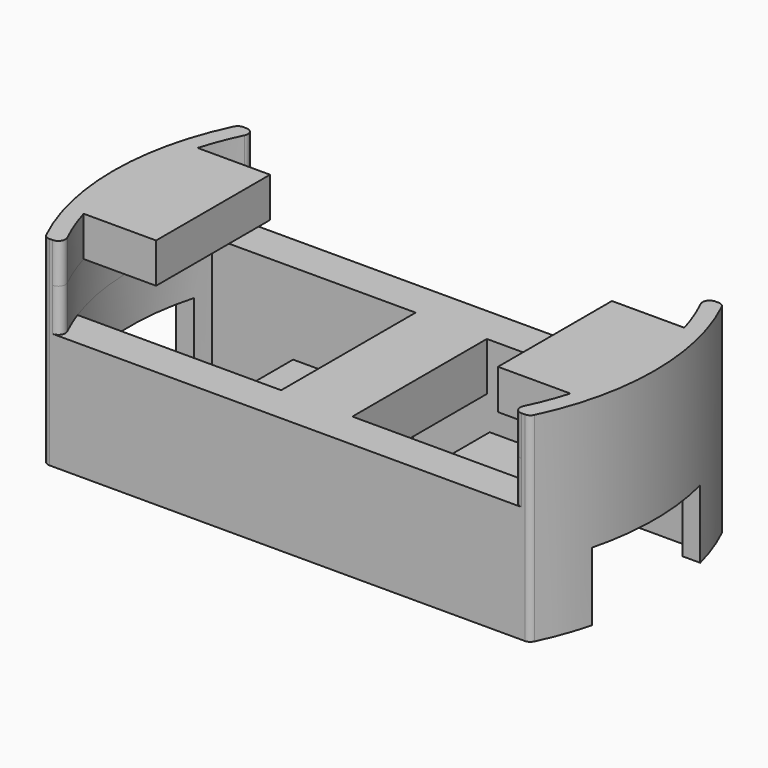
from build123d import *

# Parameters (mm, degrees)
F1_DEPTH  = 14
F2_W      = 24
F2_H      = 5.8
F3_DEPTH  = 25
F4_R      = 17.8
F4_W      = 24
F4_H      = 17
F5_DEPTH  = 3
F7_DEPTH  = 4
F9_DEPTH  = 9
F10_W     = 5
F10_H     = 11.8
F11_DEPTH = 3.4
F12_W     = 8.4
F12_H     = 3.725
F13_DEPTH = 2.5
F14_W     = 12
F14_H     = 9.5
F15_DEPTH = 4.8
F16_R     = 0.5


with BuildPart() as f1:
    # F0 (on Top) → F1 (new body)
    with BuildSketch(Plane.XY):
        with BuildLine():
            Line((-16.992645, -8.5), (16.992645, -8.5))
            ThreePointArc((16.992645, -8.5), (19, 0), (16.992645, 8.5))
            Line((16.992645, 8.5), (-16.992645, 8.5))
            ThreePointArc((-16.992645, 8.5), (-19, 0), (-16.992645, -8.5))
        make_face()
    extrude(amount=F1_DEPTH)

    # F2 (on face) → F3 (cut)
    with BuildSketch(Plane.XZ.offset(8.5)):
        with Locations((0, 11.1)):
            Rectangle(F2_W, F2_H)
    extrude(amount=-F3_DEPTH, mode=Mode.SUBTRACT)

    # F4 (on face) → F5 (cut)
    with BuildSketch(Plane.XY.offset(8.2)):
        Circle(F4_R)
        Rectangle(F4_W, F4_H, mode=Mode.SUBTRACT)
    extrude(amount=F5_DEPTH, mode=Mode.SUBTRACT)

    # F6 (on face) → F7 (cut)
    with BuildSketch(Plane.XY.offset(14)):
        with BuildLine():
            Line((12, 8.5), (15.639373, 8.5))
            ThreePointArc((15.639373, 8.5), (-1.893079, 17.699047), (-17.083325, 5))
            Line((-17.083325, 5), (12, 5))
            Line((12, 5), (12, 8.5))
        make_face()
        with BuildLine():
            Line((12, -8.5), (12, -5))
            Line((12, -5), (-17.083325, -5))
            ThreePointArc((-17.083325, -5), (-1.893079, -17.699047), (15.639373, -8.5))
            Line((15.639373, -8.5), (12, -8.5))
        make_face()
        with BuildLine():
            Line((12, 5), (17.083325, 5))
            ThreePointArc((17.083325, 5), (16.454673, 6.788501), (15.639373, 8.5))
            Line((15.639373, 8.5), (12, 8.5))
            Line((12, 8.5), (12, 5))
        make_face()
        with BuildLine():
            Line((17.083325, -5), (12, -5))
            Line((12, -5), (12, -8.5))
            Line((12, -8.5), (15.639373, -8.5))
            ThreePointArc((15.639373, -8.5), (16.454673, -6.788501), (17.083325, -5))
        make_face()
    extrude(amount=-F7_DEPTH, mode=Mode.SUBTRACT)

    # F8 (on face) → F9 (cut)
    with BuildSketch(Plane(origin=(0, 0, 0), x_dir=(1, 0, 0), z_dir=(0, 0, -1))):
        with BuildLine():
            ThreePointArc((-16.793749, 5.9), (-17.8, 0), (-16.793749, -5.9))
            Line((-16.793749, -5.9), (16.793749, -5.9))
            ThreePointArc((16.793749, -5.9), (17.8, 0), (16.793749, 5.9))
            Line((16.793749, 5.9), (-16.793749, 5.9))
        make_face()
    extrude(amount=-F9_DEPTH, mode=Mode.SUBTRACT)

    # F10 (on face) → F11 (join)
    with BuildSketch(Plane.XY.offset(8.2)):
        Rectangle(F10_W, F10_H)
    extrude(amount=-F11_DEPTH)

    # F12 (on face) → F13 (join)
    with BuildSketch(Plane(origin=(0, 0, 0), x_dir=(1, 0, 0), z_dir=(0, 0, -1))):
        with Locations((-6.9, 4.0375)):
            Rectangle(F12_W, F12_H)
        with Locations((-6.9, -4.0375)):
            Rectangle(F12_W, F12_H)
        with Locations((6.9, 4.0375)):
            Rectangle(F12_W, F12_H)
        with Locations((6.9, -4.0375)):
            Rectangle(F12_W, F12_H)
    extrude(amount=-F13_DEPTH)

    # F14 (on face) → F15 (cut)
    with BuildSketch(Plane(origin=(0, 0, 0), x_dir=(1, 0, 0), z_dir=(0, 0, -1))):
        with Locations((-18, 0)):
            Rectangle(F14_W, F14_H)
        with Locations((18, 0)):
            Rectangle(F14_W, F14_H)
    extrude(amount=-F15_DEPTH, mode=Mode.SUBTRACT)

    # F16
    f16_edges = [f1.edges().sort_by_distance(p)[0] for p in [
        (-16.992645, -8.5, 7),
        (16.992645, -8.5, 7),
        (16.992645, 8.5, 7),
        (-16.992645, 8.5, 7),
        (15.639373, -8.5, 12.6),
        (15.639373, -8.5, 10.6),
        (-15.639373, -8.5, 10.6),
        (-15.639373, -8.5, 12.6),
        (-15.639373, 8.5, 12.6),
        (-15.639373, 8.5, 10.6),
        (15.639373, 8.5, 10.6),
        (15.639373, 8.5, 12.6),
    ]]
    fillet(f16_edges, radius=F16_R)


solid = f1.part
